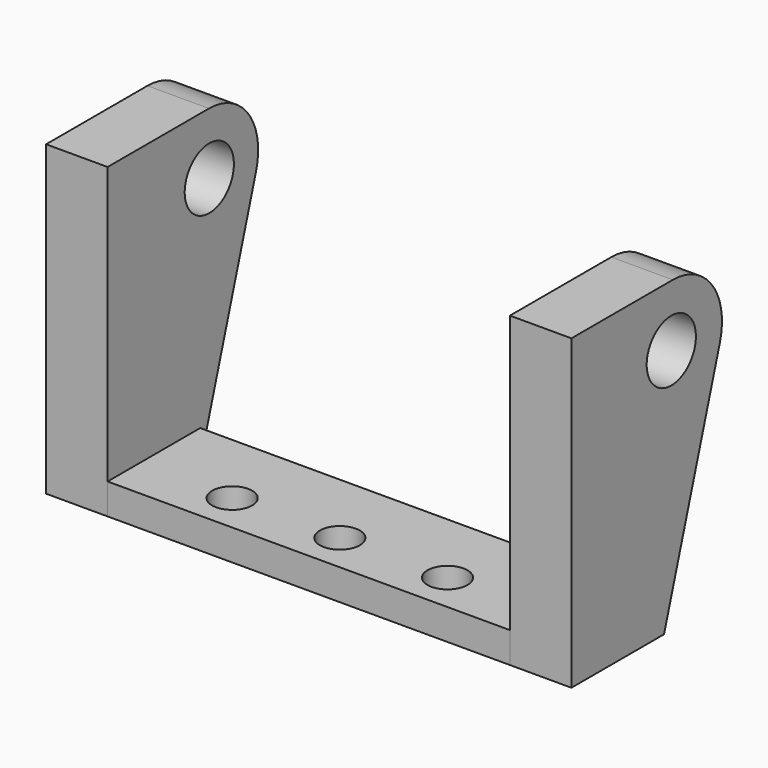
from build123d import *

# Parameters (mm, degrees)
F0_W           = 4
F0_H           = 7.5257653005
F0_H_2         = 5
F1_DEPTH       = 20
F0_W_2         = 26.1546501577
F0_R           = 1.3
F2_DEPTH       = 2
F3_SIZE2       = 16.3542630924
F3_SIZE        = 5
F4_SIZE2       = 16.3542630924
F4_SIZE        = 5
F5_R           = 2
F6_DEPTH       = 5.8
F7_R           = 2
F8_DEPTH       = 7.32
F9_T1_DEPTH    = 24
F9_2_T1_DEPTH  = 24
F10_T1_DEPTH   = 32.2377661773
F10_2_T1_DEPTH = 32.2377661773


# Not quite as in the source:
# - a fillet or chamfer that OpenCascade refuses, or shapes differently, is made with other operations: its cross-section is extruded or revolved along the edge and cut away or added


with BuildPart() as f1:
    # F0 (on Top) → F1 (new body)
    with BuildSketch(Plane.XY):
        with Locations((-14.5500070333, 7.7998988752)):
            Rectangle(F0_W, F0_H)
        with Locations((-14.5500070333, 14.0627815254)):
            Rectangle(F0_W, F0_H_2)
    extrude(amount=F1_DEPTH)

    # F3
    f3_edges = [f1.edges().sort_by_distance(p)[0] for p in [
        (-14.550007, 16.562782, 0),
    ]]
    f3_side = f1.faces().sort_by_distance((-14.550007, 10.299899, 0))[0]
    chamfer(f3_edges, length=F3_SIZE, length2=F3_SIZE2, reference=f3_side)

    # F5 (on face) → F6 (cut)
    with BuildSketch(Plane(origin=(-16.5500070333, 0, 0), x_dir=(0, -1, 0), z_dir=(-1, 0, 0))):
        with Locations((-12.2998988752, 16)):
            Circle(F5_R)
    extrude(amount=-F6_DEPTH, mode=Mode.SUBTRACT)

    # F9#2: fillet of radius 4 on 1 edges, made by hand

    # F9_2_s2 → F9_2_t1 (cut)
    with BuildSketch(Plane.YZ.offset(-26.5500070333)):
        with BuildLine():
            ThreePointArc((16.5627815254, 16), (15.3912086502, 18.8284271247), (12.5627815254, 20))
            Line((12.5627815254, 20), (16.5627815254, 20))
            Line((16.5627815254, 20), (16.5627815254, 16))
        make_face()
    extrude(amount=F9_2_T1_DEPTH, mode=Mode.SUBTRACT)

    # F10#2: fillet of radius 4 on 1 edges, made by hand

    # F10_2_s2 → F10_2_t1 (cut)
    with BuildSketch(Plane.YZ.offset(-30.668890122)):
        with BuildLine():
            ThreePointArc((12.2717054028, 20), (15.4871328453, 18.379291147), (16.0969244267, 14.8305131811))
            Line((16.0969244267, 14.8305131811), (16.479446329, 14.7135644992))
            Line((16.479446329, 14.7135644992), (16.932966821, 16.196963188))
            Line((16.932966821, 16.196963188), (16.949211258, 16.3453030569))
            ThreePointArc((16.949211258, 16.3453030569), (12.5627815254, 20.4), (12.2717054028, 20.4))
            Line((12.2717054028, 20.4), (12.2717054028, 20))
        make_face()
    extrude(amount=F10_2_T1_DEPTH, mode=Mode.SUBTRACT)


with BuildPart() as f1b:
    # F0 (on Top) → F1, piece 2 (new body)
    with BuildSketch(Plane.XY):
        with Locations((15.6046431243, 7.7998988752)):
            Rectangle(F0_W, F0_H)
        with Locations((15.6046431243, 14.0627815254)):
            Rectangle(F0_W, F0_H_2)
    extrude(amount=F1_DEPTH)

    # F4
    f4_edges = [f1b.edges().sort_by_distance(p)[0] for p in [
        (15.604643, 16.562782, 0),
    ]]
    f4_side = f1b.faces().sort_by_distance((15.604643, 10.299899, 0))[0]
    chamfer(f4_edges, length=F4_SIZE, length2=F4_SIZE2, reference=f4_side)

    # F7 (on face) → F8 (cut)
    with BuildSketch(Plane.YZ.offset(17.6046431243)):
        with Locations((12.1530162249, 16)):
            Circle(F7_R)
    extrude(amount=-F8_DEPTH, mode=Mode.SUBTRACT)

    # F9: fillet of radius 4 on 1 edges, made by hand

    # F9_s2 → F9_t1 (cut)
    with BuildSketch(Plane.YZ.offset(3.6046431243)):
        with BuildLine():
            ThreePointArc((16.5627815254, 16), (15.3912086502, 18.8284271247), (12.5627815254, 20))
            Line((12.5627815254, 20), (16.5627815254, 20))
            Line((16.5627815254, 20), (16.5627815254, 16))
        make_face()
    extrude(amount=F9_T1_DEPTH, mode=Mode.SUBTRACT)

    # F10: fillet of radius 4 on 1 edges, made by hand

    # F10_s2 → F10_t1 (cut)
    with BuildSketch(Plane.YZ.offset(-0.5142399643)):
        with BuildLine():
            ThreePointArc((12.2717054028, 20), (15.4871328453, 18.379291147), (16.0969244267, 14.8305131811))
            Line((16.0969244267, 14.8305131811), (16.479446329, 14.7135644992))
            Line((16.479446329, 14.7135644992), (16.932966821, 16.196963188))
            Line((16.932966821, 16.196963188), (16.949211258, 16.3453030569))
            ThreePointArc((16.949211258, 16.3453030569), (12.5627815254, 20.4), (12.2717054028, 20.4))
            Line((12.2717054028, 20.4), (12.2717054028, 20))
        make_face()
    extrude(amount=F10_T1_DEPTH, mode=Mode.SUBTRACT)


with BuildPart() as f2:
    # F0 (on Top) → F2 (new body)
    with BuildSketch(Plane.XY):
        with Locations((0.5273180455, 7.7998988752)):
            Rectangle(F0_W_2, F0_H)
        with Locations((-6.4726819545, 6.5627815254)):
            Circle(F0_R, mode=Mode.SUBTRACT)
        with Locations((0.5273180455, 6.5627815254)):
            Circle(F0_R, mode=Mode.SUBTRACT)
        with Locations((7.5273180455, 6.5627815254)):
            Circle(F0_R, mode=Mode.SUBTRACT)
    extrude(amount=F2_DEPTH)


solid = Compound([f1.part, f1b.part, f2.part])
